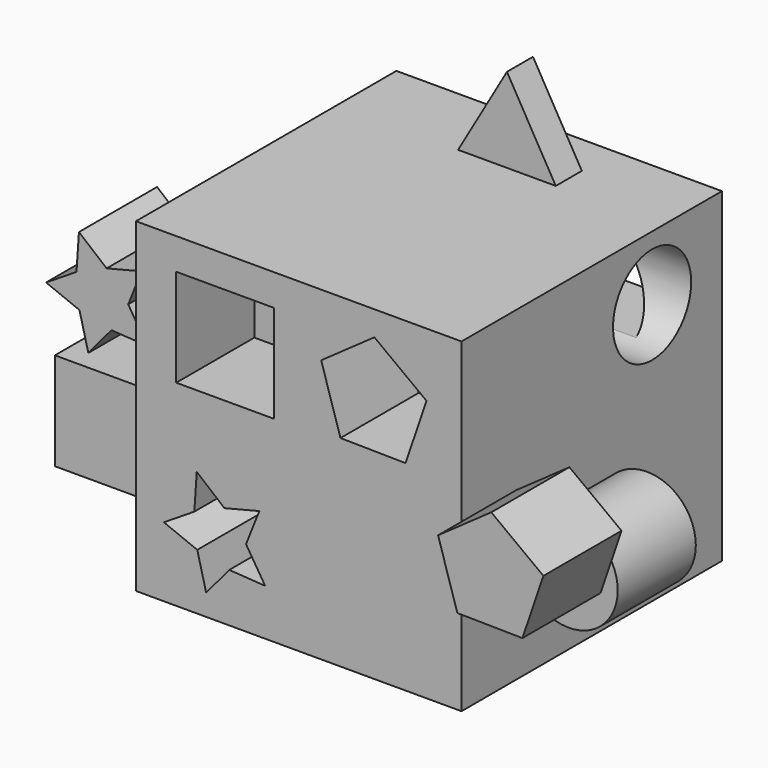
from build123d import *

# Parameters (mm, degrees)
F0_W      = 127
F0_H      = 127
F1_DEPTH  = 63.5
F2_W      = 38.1
F2_H      = 38.1
F3_DEPTH  = 38.1
F5_DEPTH  = 38.1
F7_DEPTH  = 38.1
F8_R      = 19.05
F9_DEPTH  = 38.1
F11_DEPTH = 38.1
F12_R     = 19.05
F13_DEPTH = 38.1
F15_DEPTH = 38.1
F16_W     = 38.1
F16_H     = 38.1
F17_DEPTH = 38.1
F18_R     = 19.05
F19_DEPTH = 38.1
F21_DEPTH = 38.1
F24_DEPTH = 12.7


# Not quite as in the source:
# - the program builds the solid bodies; features that only make, move or delete a surface that nothing else refers to are left out


with BuildPart() as f1:
    # F0 (on Front) → F1 (new body, symmetric)
    with BuildSketch(Plane.XZ):
        Rectangle(F0_W, F0_H)
    extrude(amount=F1_DEPTH, both=True)

    # F2 (on face) → F3 (cut)
    with BuildSketch(Plane.XZ.offset(63.5)):
        with Locations((-28.7386754062, 32.1922943337)):
            Rectangle(F2_W, F2_H)
        with Locations((86.2550362945, -6.9399550557)):
            Rectangle(F2_W, F2_H)
    extrude(amount=-F3_DEPTH, mode=Mode.SUBTRACT)

    # F4 (on face) → F5 (cut)
    with BuildSketch(Plane.XZ.offset(63.5)):
        Polygon((8.7614915837, 39.2321395601), (16.2751341757, 14.9688921476), (41.6726969844, 14.6170351066), (49.8556114396, 38.6628229086), (29.5153678912, 53.8757940975), align=None)
    extrude(amount=-F5_DEPTH, mode=Mode.SUBTRACT)

    # F6 (on face) → F7 (cut)
    with BuildSketch(Plane(origin=(0, 63.5, 0), x_dir=(-1, 0, 0), z_dir=(0, 1, 0))):
        Polygon((-51.8942007303, 20.5241581157), (-13.7942007303, 20.5241581157), (-32.8442007303, 53.5197259999), align=None)
    extrude(amount=-F7_DEPTH, mode=Mode.SUBTRACT)

    # F8 (on face) → F9 (cut)
    with BuildSketch(Plane(origin=(0, 63.5, 0), x_dir=(-1, 0, 0), z_dir=(0, 1, 0))):
        with Locations((24.542177096, 34.7635373473)):
            Circle(F8_R)
    extrude(amount=-F9_DEPTH, mode=Mode.SUBTRACT)

    # F10 (on face) → F11 (cut)
    with BuildSketch(Plane.XZ.offset(63.5)):
        Polygon((-39.7797108135, -14.8606818497), (-40.7370848933, -28.8630111208), (-52.6019230047, -36.3601710319), (-39.5807613688, -41.5976455947), (-36.1169751935, -55.1985270174), (-27.1120806497, -44.4331350413), (-13.1065049523, -45.3417821264), (-20.5623356949, -33.4509294202), (-15.3702000572, -20.4116227799), (-28.9830514143, -23.8280636283), align=None)
    extrude(amount=-F11_DEPTH, mode=Mode.SUBTRACT)

    # F12 (on face) → F13 (cut)
    with BuildSketch(Plane.YZ.offset(63.5)):
        with Locations((29.4494424015, 38.3474603295)):
            Circle(F12_R)
    extrude(amount=-F13_DEPTH, mode=Mode.SUBTRACT)


with BuildPart() as f15:
    # F14 (on face) → F15 (new body)
    with BuildSketch(Plane.XZ.offset(63.5)):
        Polygon((84.8394576032, 19.3606587971), (92.3531001952, -4.9025886154), (117.7506630039, -5.2544456563), (125.9335774591, 18.7913421457), (105.5933339107, 34.0043133345), align=None)
    extrude(amount=F15_DEPTH)


with BuildPart() as f17:
    # F16 (on Front) → F17 (new body)
    with BuildSketch(Plane.XZ):
        with Locations((-96.3894203305, -28.8341529667)):
            Rectangle(F16_W, F16_H)
    extrude(amount=F17_DEPTH)


with BuildPart() as f19:
    # F18 (on Front) → F19 (new body)
    with BuildSketch(Plane.XZ):
        with Locations((85.0661173463, -19.0954655409)):
            Circle(F18_R)
    extrude(amount=F19_DEPTH)


with BuildPart() as f21:
    # F20 (on Front) → F21 (new body)
    with BuildSketch(Plane.XZ):
        Polygon((-106.0621396145, 35.6140661657), (-107.0195136944, 21.6117368946), (-118.8843518057, 14.1145769835), (-105.8631901699, 8.8771024207), (-102.3994039946, -4.723779002), (-93.3945094508, 6.0416129741), (-79.3889337533, 5.132965889), (-86.844764496, 17.0238185952), (-81.6526288582, 30.0631252355), (-95.2654802154, 26.6466843871), align=None)
    extrude(amount=F21_DEPTH)


with BuildPart() as f24:
    # F22 (on Front) → F24 (new body)
    with BuildSketch(Plane.XZ):
        Polygon((21.5419738114, 95.014536988), (59.6419738114, 95.014536988), (40.5919738114, 128.0101048722), align=None)
    extrude(amount=F24_DEPTH)


solid = Compound([f1.part, f15.part, f17.part, f19.part, f21.part, f24.part])
